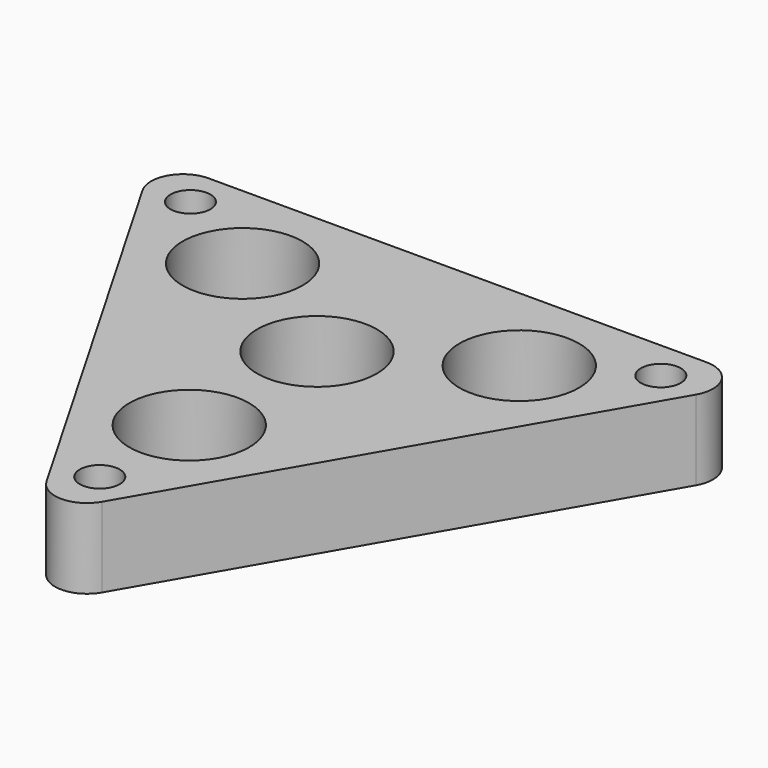
from build123d import *

# Parameters (mm, degrees)
F0_R     = 1.5875
F0_R_2   = 4.7625
F1_DEPTH = 6.35
F2_R     = 2.54


# Not quite as in the source:
# - a length typed as a fraction of an inch, garbled in the dataset ("3 / 203.2 mm" for 3/8 in), is restored


with BuildPart() as f1:
    # F0 (on Top) → F1 (new body)
    with BuildSketch(Plane.XY):
        Polygon((-24.1967497817, 13.97), (0, -27.94), (24.1967497817, 13.97), align=None)
        with Locations((0, -21.59)):
            Circle(F0_R, mode=Mode.SUBTRACT)
        with Locations((0, -12.7)):
            Circle(F0_R_2, mode=Mode.SUBTRACT)
        Circle(F0_R_2, mode=Mode.SUBTRACT)
        with Locations((-18.6974884677, 10.795)):
            Circle(F0_R, mode=Mode.SUBTRACT)
        with Locations((-10.9985226281, 6.35)):
            Circle(F0_R_2, mode=Mode.SUBTRACT)
        with Locations((10.9985226281, 6.35)):
            Circle(F0_R_2, mode=Mode.SUBTRACT)
        with Locations((18.6974884677, 10.795)):
            Circle(F0_R, mode=Mode.SUBTRACT)
    extrude(amount=F1_DEPTH)

    # F2
    f2_edges = [f1.edges().sort_by_distance(p)[0] for p in [
        (-24.19675, 13.97, 3.175),
        (0, -27.94, 3.175),
        (24.19675, 13.97, 3.175),
    ]]
    fillet(f2_edges, radius=F2_R)


solid = f1.part
